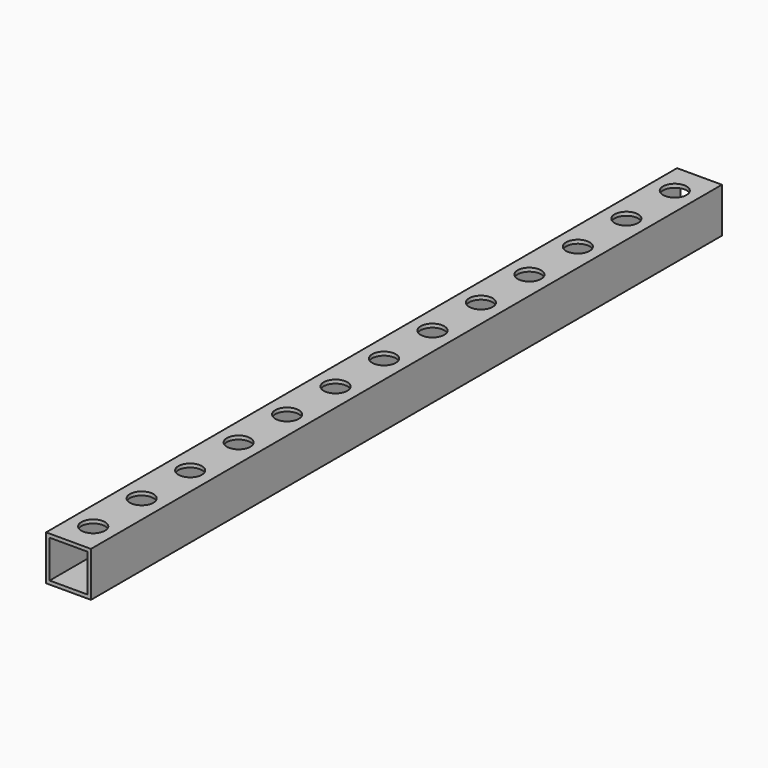
from build123d import *

# Parameters (mm, degrees)
F0_W     = 20
F0_H     = 20
F0_W_2   = 16.8
F0_H_2   = 16.8
F1_DEPTH = 351.5
F2_R     = 5.25
F3_DEPTH = 5


# Not quite as in the source:
# - a feature names something its author has since deleted; it is built from what else it names


with BuildPart() as f1:
    # F0 (on Front) → F1 (new body)
    with BuildSketch(Plane.XZ):
        with Locations((10, -10)):
            Rectangle(F0_W, F0_H)
        with Locations((10, -10)):
            Rectangle(F0_W_2, F0_H_2, mode=Mode.SUBTRACT)
    extrude(amount=F1_DEPTH)

    # F2 (on face) → F3 (cut)
    with BuildSketch(Plane.XY):
        with Locations((10, -310.75)):
            Circle(F2_R)
        with Locations((10, -283.75)):
            Circle(F2_R)
        with Locations((10, -256.75)):
            Circle(F2_R)
        with Locations((10, -229.75)):
            Circle(F2_R)
        with Locations((10, -202.75)):
            Circle(F2_R)
        with Locations((10, -175.75)):
            Circle(F2_R)
        with Locations((10, -148.75)):
            Circle(F2_R)
        with Locations((10, -121.75)):
            Circle(F2_R)
        with Locations((10, -94.75)):
            Circle(F2_R)
        with Locations((10, -67.75)):
            Circle(F2_R)
        with Locations((10, -40.75)):
            Circle(F2_R)
        with Locations((10, -13.75)):
            Circle(F2_R)
        with Locations((10, -337.75)):
            Circle(F2_R)
    extrude(amount=-F3_DEPTH, mode=Mode.SUBTRACT)


solid = f1.part
